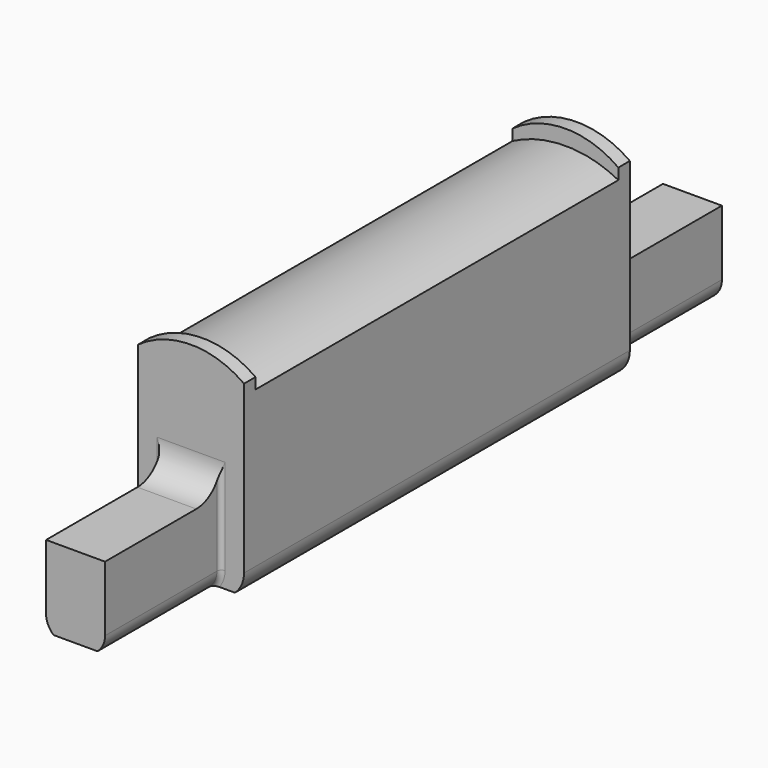
from build123d import *

# Parameters (mm, degrees)
F1_DEPTH = 40.513
F2_DEPTH = 38.1
F3_DEPTH = 64.77
F5_R     = 5.08
F6_R     = 0.762


with BuildPart() as f1:
    # F0 (on Front) → F1 (new body)
    with BuildSketch(Plane.XZ):
        with BuildLine():
            Line((8.89, 22.7287972945), (8.89, 24.5818064272))
            Line((8.89, 24.5818064272), (3.5665511583, 24.5818064272))
            ThreePointArc((3.5665511583, 24.5818064272), (6.2968108914, 23.8521946995), (8.89, 22.7287972945))
        make_face()
        with BuildLine():
            Line((3.5665511583, 24.5818064272), (8.89, 24.5818064272))
            ThreePointArc((8.89, 24.5818064272), (0, 27.4567800376), (-8.89, 24.5818064272))
            Line((-8.89, 24.5818064272), (-3.5665511583, 24.5818064272))
            ThreePointArc((-3.5665511583, 24.5818064272), (0, 24.9167800376), (3.5665511583, 24.5818064272))
        make_face()
        with BuildLine():
            ThreePointArc((8.89, 22.7287972945), (6.2968108914, 23.8521946995), (3.5665511583, 24.5818064272))
            Line((3.5665511583, 24.5818064272), (-3.5665511583, 24.5818064272))
            ThreePointArc((-3.5665511583, 24.5818064272), (-6.2968108914, 23.8521946995), (-8.89, 22.7287972945))
            Line((-8.89, 22.7287972945), (8.89, 22.7287972945))
        make_face()
        with BuildLine():
            Line((-3.5665511583, 24.5818064272), (3.5665511583, 24.5818064272))
            ThreePointArc((3.5665511583, 24.5818064272), (0, 24.9167800376), (-3.5665511583, 24.5818064272))
        make_face()
        with BuildLine():
            Line((8.89, -3.4254523647), (8.89, 22.7287972945))
            Line((8.89, 22.7287972945), (-8.89, 22.7287972945))
            Line((-8.89, 22.7287972945), (-8.89, -3.4254523647))
            ThreePointArc((-8.89, -3.4254523647), (-8.4916458882, -5.2919635487), (-7.366, -6.8332199624))
            Line((-7.366, -6.8332199624), (-4.953, -6.8332199624))
            Line((-4.953, -6.8332199624), (-4.953, -4.1093734175))
            Line((-4.953, -4.1093734175), (-4.953, 0))
            Line((-4.953, 0), (-4.953, 6.8332199624))
            Line((-4.953, 6.8332199624), (4.953, 6.8332199624))
            Line((4.953, 6.8332199624), (4.953, 0))
            Line((4.953, 0), (4.953, -4.1093734175))
            Line((4.953, -4.1093734175), (4.953, -6.8332199624))
            Line((4.953, -6.8332199624), (7.366, -6.8332199624))
            ThreePointArc((7.366, -6.8332199624), (8.4916458882, -5.2919635487), (8.89, -3.4254523647))
        make_face()
        with BuildLine():
            Line((-3.5665511583, 24.5818064272), (-8.89, 24.5818064272))
            Line((-8.89, 24.5818064272), (-8.89, 22.7287972945))
            ThreePointArc((-8.89, 22.7287972945), (-6.2968108914, 23.8521946995), (-3.5665511583, 24.5818064272))
        make_face()
        with BuildLine():
            Line((3.683, -6.8332199624), (4.953, -6.8332199624))
            Line((4.953, -6.8332199624), (4.953, -4.1093734175))
            ThreePointArc((4.953, -4.1093734175), (4.6198986953, -5.6120576825), (3.683, -6.8332199624))
        make_face()
        with BuildLine():
            Line((-3.683, -6.8332199624), (3.683, -6.8332199624))
            ThreePointArc((3.683, -6.8332199624), (4.6198986953, -5.6120576825), (4.953, -4.1093734175))
            Line((4.953, -4.1093734175), (4.953, 0))
            ThreePointArc((4.953, 0), (0, -4.953), (-4.953, 0))
            Line((-4.953, 0), (-4.953, -4.1093734175))
            ThreePointArc((-4.953, -4.1093734175), (-4.6198986953, -5.6120576825), (-3.683, -6.8332199624))
        make_face()
        with BuildLine():
            Line((-4.953, -4.1093734175), (-4.953, -6.8332199624))
            Line((-4.953, -6.8332199624), (-3.683, -6.8332199624))
            ThreePointArc((-3.683, -6.8332199624), (-4.6198986953, -5.6120576825), (-4.953, -4.1093734175))
        make_face()
        with BuildLine():
            ThreePointArc((-4.953, 0), (0, -4.953), (4.953, 0))
            ThreePointArc((4.953, 0), (0, 4.953), (-4.953, 0))
        make_face()
        with BuildLine():
            ThreePointArc((-4.953, 0), (0, 4.953), (4.953, 0))
            Line((4.953, 0), (4.953, 6.8332199624))
            Line((4.953, 6.8332199624), (-4.953, 6.8332199624))
            Line((-4.953, 6.8332199624), (-4.953, 0))
        make_face()
    extrude(amount=F1_DEPTH)

    # F0 (on Front) → F2 (cut)
    with BuildSketch(Plane.XZ):
        with BuildLine():
            Line((-3.5665511583, 24.5818064272), (-8.89, 24.5818064272))
            Line((-8.89, 24.5818064272), (-8.89, 22.7287972945))
            ThreePointArc((-8.89, 22.7287972945), (-6.2968108914, 23.8521946995), (-3.5665511583, 24.5818064272))
        make_face()
        with BuildLine():
            Line((3.5665511583, 24.5818064272), (8.89, 24.5818064272))
            ThreePointArc((8.89, 24.5818064272), (0, 27.4567800376), (-8.89, 24.5818064272))
            Line((-8.89, 24.5818064272), (-3.5665511583, 24.5818064272))
            ThreePointArc((-3.5665511583, 24.5818064272), (0, 24.9167800376), (3.5665511583, 24.5818064272))
        make_face()
        with BuildLine():
            Line((8.89, 22.7287972945), (8.89, 24.5818064272))
            Line((8.89, 24.5818064272), (3.5665511583, 24.5818064272))
            ThreePointArc((3.5665511583, 24.5818064272), (6.2968108914, 23.8521946995), (8.89, 22.7287972945))
        make_face()
    extrude(amount=F2_DEPTH, mode=Mode.SUBTRACT)

    # F0 (on Front) → F3 (join)
    with BuildSketch(Plane.XZ):
        with BuildLine():
            Line((-3.683, -6.8332199624), (3.683, -6.8332199624))
            ThreePointArc((3.683, -6.8332199624), (4.6198986953, -5.6120576825), (4.953, -4.1093734175))
            Line((4.953, -4.1093734175), (4.953, 0))
            ThreePointArc((4.953, 0), (0, -4.953), (-4.953, 0))
            Line((-4.953, 0), (-4.953, -4.1093734175))
            ThreePointArc((-4.953, -4.1093734175), (-4.6198986953, -5.6120576825), (-3.683, -6.8332199624))
        make_face()
        with BuildLine():
            ThreePointArc((-4.953, 0), (0, -4.953), (4.953, 0))
            ThreePointArc((4.953, 0), (0, 4.953), (-4.953, 0))
        make_face()
        with BuildLine():
            ThreePointArc((-4.953, 0), (0, 4.953), (4.953, 0))
            Line((4.953, 0), (4.953, 6.8332199624))
            Line((4.953, 6.8332199624), (-4.953, 6.8332199624))
            Line((-4.953, 6.8332199624), (-4.953, 0))
        make_face()
    extrude(amount=F3_DEPTH)

    # F4: F1 across plane


with BuildPart() as f1_1:
    add(f1.part)
    add(f1.part.mirror(Plane.XZ))

    # F5
    f5_edges = [f1_1.edges().sort_by_distance(p)[0] for p in [
        (0, -40.513, 6.83322),
        (0, 40.513, 6.83322),
    ]]
    fillet(f5_edges, radius=F5_R)

    # F6
    f6_edges = [f1_1.edges().sort_by_distance(p)[0] for p in [
        (-4.953, 40.513, 1.361923),
        (-4.619899, 40.513, -5.612058),
        (-4.953, -40.513, 1.361923),
        (-4.619899, -40.513, -5.612058),
        (4.619899, -40.513, -5.612058),
        (4.953, -40.513, 1.361923),
        (4.953, 40.513, 1.361923),
        (4.619899, 40.513, -5.612058),
        (-4.953, 40.513, 9.37322),
        (4.953, 40.513, 9.37322),
        (-4.953, -40.513, 9.37322),
        (4.953, -40.513, 9.37322),
    ]]
    fillet(f6_edges, radius=F6_R)


solid = f1_1.part
